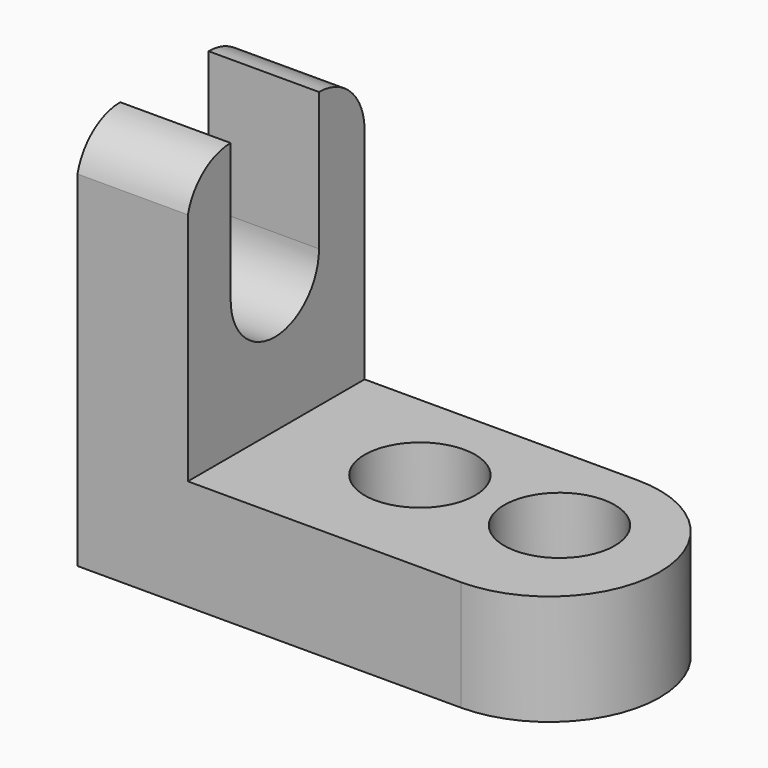
from build123d import *

# Parameters (mm, degrees)
F1_DEPTH = 25.4
F3_DEPTH = 12.7
F4_R     = 6.35
F5_DEPTH = 12.7


with BuildPart() as f1:
    # F0 (on Front) → F1 (new body)
    with BuildSketch(Plane.XZ):
        Polygon((0, 44.45), (0, 0), (57.15, 0), (57.15, 12.7), (12.7, 12.7), (12.7, 44.45), align=None)
    extrude(amount=F1_DEPTH)

    # F2 (on face) → F3 (cut)
    with BuildSketch(Plane.YZ.offset(12.7)):
        with BuildLine():
            ThreePointArc((-19.2516389379, 28.575), (-12.9016389379, 22.225), (-6.5516389379, 28.575))
            ThreePointArc((-6.5516389379, 28.575), (-12.9016389379, 34.925), (-19.2516389379, 28.575))
        make_face()
        with BuildLine():
            ThreePointArc((-19.2516389379, 28.575), (-12.9016389379, 34.925), (-6.5516389379, 28.575))
            Line((-6.5516389379, 28.575), (-6.5516389379, 44.45))
            Line((-6.5516389379, 44.45), (-19.2516389379, 44.45))
            Line((-19.2516389379, 44.45), (-19.2516389379, 28.575))
        make_face()
        with BuildLine():
            Line((0, 44.45), (-6.5516389379, 44.45))
            ThreePointArc((-6.5516389379, 44.45), (-1.9896636866, 42.6019965832), (0, 38.1))
            Line((0, 38.1), (0, 44.45))
        make_face()
        with BuildLine():
            ThreePointArc((-25.4, 39.6875), (-23.1402039046, 43.1201157855), (-19.2516389379, 44.45))
            Line((-19.2516389379, 44.45), (-25.4, 44.45))
            Line((-25.4, 44.45), (-25.4, 39.6875))
        make_face()
    extrude(amount=-F3_DEPTH, mode=Mode.SUBTRACT)

    # F4 (on face) → F5 (cut)
    with BuildSketch(Plane.XY.offset(12.7)):
        with Locations((28.2040209995, -11.4295053813)):
            Circle(F4_R)
        with Locations((44.1000172256, -11.2356515601)):
            Circle(F4_R)
        with BuildLine():
            ThreePointArc((44.1000172256, 0), (56.8000172256, -12.7), (44.1000172256, -25.4))
            Line((44.1000172256, -25.4), (57.15, -25.4))
            Line((57.15, -25.4), (57.15, 0))
            Line((57.15, 0), (44.1000172256, 0))
        make_face()
    extrude(amount=-F5_DEPTH, mode=Mode.SUBTRACT)


solid = f1.part
